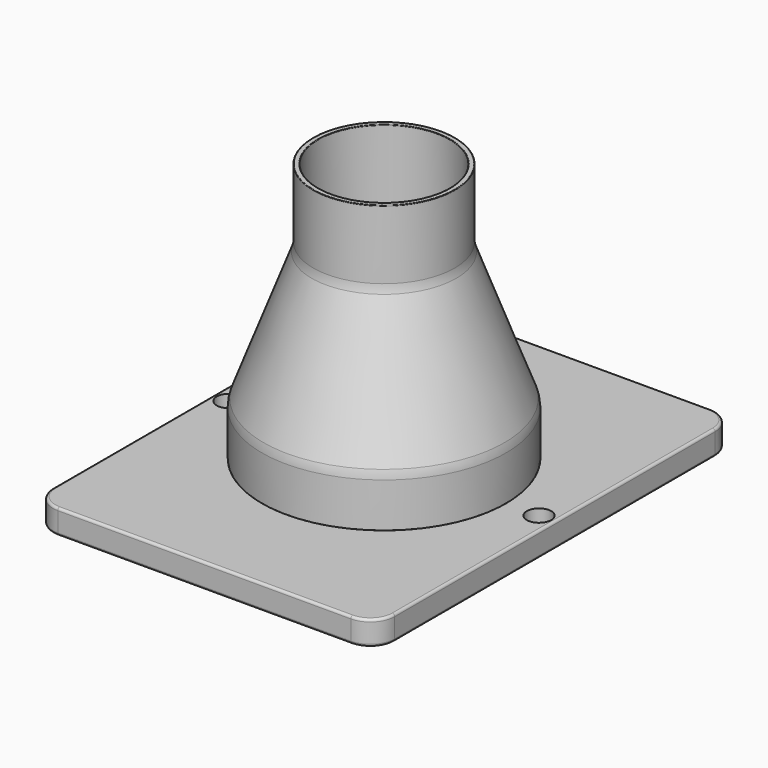
from build123d import *

# Parameters (mm, degrees)
F2_W         = 70
F2_H         = 92
F2_R         = 25
F3_DEPTH     = 5
F4_R         = 2.5
F5_DEPTH     = 25
F6_T1_DEPTH  = 94.5
F6_T3_DEPTH  = 72.5
F7_T1_DEPTH  = 17.5
F7_T4_ANGLE  = 90
F7_T6_ANGLE  = 90
F7_T8_ANGLE  = 90
F7_T10_ANGLE = 90
F8_R         = 0.5
F9_R         = 5
F10_R        = 0.1


# Not quite as in the source:
# - a fillet or chamfer that OpenCascade refuses, or shapes differently, is made with other operations: its cross-section is extruded or revolved along the edge and cut away or added


with BuildPart() as f1:
    # F0 (on Front) → F1 (revolve)
    with BuildSketch(Plane.XZ):
        Polygon((-25, 10), (-25, 0), (-24, 0), (-24, 9.8192848565), (-13.5, 37.9217758492), (-13.5, 53.1024909928), (-14.5, 53.1024909928), (-14.5, 38.1024909928), align=None)
    revolve(axis=Axis((0, 0, 23.4480407089), (0, 0, 1)))

    # F9
    f9_edges = [f1.edges().sort_by_distance(p)[0] for p in [
        (25, 0, 10),
        (14.5, 0, 38.102491),
    ]]
    fillet(f9_edges, radius=F9_R)

    # F10
    f10_edges = [f1.edges().sort_by_distance(p)[0] for p in [
        (13.5, 0, 53.102491),
        (14.5, 0, 53.102491),
    ]]
    fillet(f10_edges, radius=F10_R)


with BuildPart() as f3:
    # F2 (on face) → F3 (new body)
    with BuildSketch(Plane(origin=(0, 0, 0), x_dir=(1, 0, 0), z_dir=(0, 0, -1))):
        Rectangle(F2_W, F2_H)
        Circle(F2_R, mode=Mode.SUBTRACT)
    extrude(amount=F3_DEPTH)

    # F4 (on face) → F5 (cut)
    with BuildSketch(Plane(origin=(0, 0, -5), x_dir=(1, 0, 0), z_dir=(0, 0, -1))):
        with Locations((-31.75, 0)):
            Circle(F4_R)
        with Locations((31.75, 0)):
            Circle(F4_R)
    extrude(amount=-F5_DEPTH, mode=Mode.SUBTRACT)

    # F6: fillet of radius 0.5 on 7 edges, made by hand

    # F6_s2 → F6_t1 (cut)
    with BuildSketch(Plane.XZ.offset(-47.25)):
        with BuildLine():
            ThreePointArc((35, -4.5), (34.8535533906, -4.8535533906), (34.5, -5))
            Line((34.5, -5), (35, -5))
            Line((35, -5), (35, -4.5))
        make_face()
        with BuildLine():
            ThreePointArc((-34.5, -5), (-34.8535533906, -4.8535533906), (-35, -4.5))
            Line((-35, -4.5), (-35, -5))
            Line((-35, -5), (-34.5, -5))
        make_face()
    extrude(amount=F6_T1_DEPTH, mode=Mode.SUBTRACT)

    # F6_s4 → F6_t3 (cut)
    with BuildSketch(Plane.YZ.offset(-36.25)):
        with BuildLine():
            ThreePointArc((46, -4.5), (45.8535533906, -4.8535533906), (45.5, -5))
            Line((45.5, -5), (46, -5))
            Line((46, -5), (46, -4.5))
        make_face()
        with BuildLine():
            ThreePointArc((-46, -4.5), (-45.8535533906, -4.8535533906), (-45.5, -5))
            Line((-45.5, -5), (-46, -5))
            Line((-46, -5), (-46, -4.5))
        make_face()
    extrude(amount=F6_T3_DEPTH, mode=Mode.SUBTRACT)

    # F6_s5 → F6_t6 (revolve, cut)
    with BuildSketch(Plane.XZ):
        with BuildLine():
            ThreePointArc((-28.75, -5), (-29.1035533906, -4.8535533906), (-29.25, -4.5))
            Line((-29.25, -4.5), (-29.25, -5))
            Line((-29.25, -5), (-28.75, -5))
        make_face()
    revolve(axis=Axis((-31.75, 0, -5), (0, 0, -1)), mode=Mode.SUBTRACT)

    # F6_s7 → F6_t8 (revolve, cut)
    with BuildSketch(Plane.XZ):
        with BuildLine():
            ThreePointArc((25.5, -5), (25.1464466094, -4.8535533906), (25, -4.5))
            Line((25, -4.5), (25, -5))
            Line((25, -5), (25.5, -5))
        make_face()
    revolve(axis=Axis((0, 0, -5), (0, 0, -1)), mode=Mode.SUBTRACT)

    # F6_s9 → F6_t10 (revolve, cut)
    with BuildSketch(Plane.XZ):
        with BuildLine():
            ThreePointArc((34.75, -5), (34.3964466094, -4.8535533906), (34.25, -4.5))
            Line((34.25, -4.5), (34.25, -5))
            Line((34.25, -5), (34.75, -5))
        make_face()
    revolve(axis=Axis((31.75, 0, -5), (0, 0, -1)), mode=Mode.SUBTRACT)

    # F7: fillet of radius 5 on 4 edges, made by hand

    # F7_s2 → F7_t1 (cut)
    with BuildSketch(Plane.XY.offset(-5)):
        with BuildLine():
            ThreePointArc((35, -41), (33.5355339059, -44.5355339059), (30, -46))
            Line((30, -46), (35, -46))
            Line((35, -46), (35, -41))
        make_face()
        with BuildLine():
            ThreePointArc((35, 41), (33.5355339059, 44.5355339059), (30, 46))
            Line((30, 46), (35, 46))
            Line((35, 46), (35, 41))
        make_face()
        with BuildLine():
            ThreePointArc((-30, -46), (-33.5355339059, -44.5355339059), (-35, -41))
            Line((-35, -41), (-35, -46))
            Line((-35, -46), (-30, -46))
        make_face()
        with BuildLine():
            ThreePointArc((-30, 46), (-33.5355339059, 44.5355339059), (-35, 41))
            Line((-35, 41), (-35, 46))
            Line((-35, 46), (-30, 46))
        make_face()
    extrude(amount=F7_T1_DEPTH, mode=Mode.SUBTRACT)

    # F7_s3 → F7_t4 (revolve, cut)
    with BuildSketch(Plane.XZ.offset(-41)):
        with BuildLine():
            ThreePointArc((-34.5, -5), (-34.8535533906, -4.8535533906), (-35, -4.5))
            Line((-35, -4.5), (-35, -5))
            Line((-35, -5), (-34.5, -5))
        make_face()
    revolve(axis=Axis((-30, 41, -5), (0, 0, -1)), revolution_arc=F7_T4_ANGLE, mode=Mode.SUBTRACT)

    # F7_s5 → F7_t6 (revolve, cut)
    with BuildSketch(Plane.YZ.offset(-30)):
        with BuildLine():
            ThreePointArc((-45.5, -5), (-45.8535533906, -4.8535533906), (-46, -4.5))
            Line((-46, -4.5), (-46, -5))
            Line((-46, -5), (-45.5, -5))
        make_face()
    revolve(axis=Axis((-30, -41, -5), (0, 0, -1)), revolution_arc=F7_T6_ANGLE, mode=Mode.SUBTRACT)

    # F7_s7 → F7_t8 (revolve, cut)
    with BuildSketch(Plane.YZ.offset(30)):
        with BuildLine():
            ThreePointArc((45.5, -5), (45.8535533906, -4.8535533906), (46, -4.5))
            Line((46, -4.5), (46, -5))
            Line((46, -5), (45.5, -5))
        make_face()
    revolve(axis=Axis((30, 41, -5), (0, 0, -1)), revolution_arc=F7_T8_ANGLE, mode=Mode.SUBTRACT)

    # F7_s9 → F7_t10 (revolve, cut)
    with BuildSketch(Plane.XZ.offset(41)):
        with BuildLine():
            ThreePointArc((34.5, -5), (34.8535533906, -4.8535533906), (35, -4.5))
            Line((35, -4.5), (35, -5))
            Line((35, -5), (34.5, -5))
        make_face()
    revolve(axis=Axis((30, -41, -5), (0, 0, -1)), revolution_arc=F7_T10_ANGLE, mode=Mode.SUBTRACT)

    # F8
    f8_edges = [f3.edges().sort_by_distance(p)[0] for p in [
        (0, -46, 0),
        (35, 0, 0),
        (33.535534, 44.535534, 0),
        (0, 46, 0),
        (-33.535534, 44.535534, 0),
        (-35, 0, 0),
        (-33.535534, -44.535534, 0),
        (33.535534, -44.535534, 0),
    ]]
    fillet(f8_edges, radius=F8_R)


solid = Compound([f1.part, f3.part])
